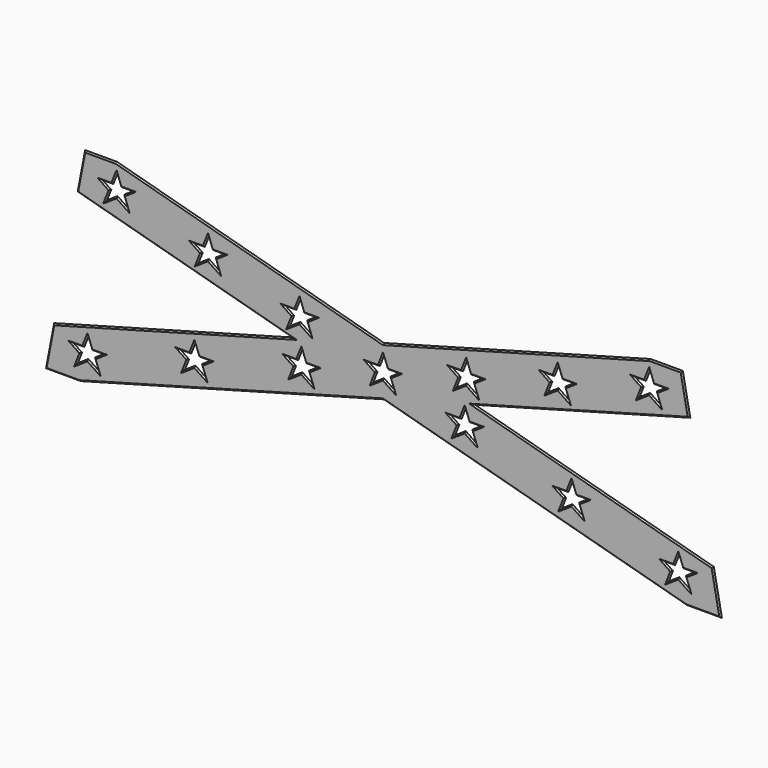
from build123d import *

# Parameters (mm, degrees)
F2_DEPTH = 3.175
F4_DEPTH = 3.175
F5_SIZE  = 3.17499


# Not quite as in the source:
# - a fillet or chamfer is up to 0.001 mm smaller than in the source, because OpenCascade refuses the exact size


with BuildPart() as f2:
    # F1 (on face) → F2 (new body)
    with BuildSketch(Plane.XZ):
        Polygon((-719.0774731079, 243.080791305), (-736.9299944829, 149.538113026), (-219.4252927257, 8.6387051816), (-793.6587311705, -147.7060607049), (-813.1201987879, -249.679208695), (-729.3418953294, -249.679208695), (0, -51.1035420022), (729.3418953294, -249.679208695), (813.1201987879, -249.679208695), (793.6587311705, -147.7060607049), (219.4252927257, 8.6387051816), (736.9299944829, 149.538113026), (719.0774731079, 243.080791305), (641.6491696493, 243.080791305), (0, 68.3809523654), (-641.6491696493, 243.080791305), align=None)
    extrude(amount=F2_DEPTH)

    # F3 (on face) → F4 (cut)
    with BuildSketch(Plane.XZ.offset(3.175)):
        Polygon((-641.1379151514, 218.6439759686), (-651.400474936, 193.2439759686), (-676.8718986419, 193.2439759686), (-656.2753553668, 179.4930621766), (-666.5379151514, 154.0930621766), (-641.1379151514, 171.0509179514), (-615.7379151514, 154.0930621766), (-625.1066068913, 179.4930621766), (-604.5100636162, 193.2439759686), (-631.7692234114, 193.2439759686), align=None)
        Polygon((-436.1568656837, 117.8018107739), (-446.4194254683, 92.4018107739), (-421.0194254683, 109.3596665488), (-395.6194254683, 92.4018107739), (-404.9881172082, 117.8018107739), (-384.3915739331, 131.552724566), (-411.6507337283, 131.552724566), (-421.0194254683, 156.952724566), (-431.2819852529, 131.552724566), (-456.7534089588, 131.552724566), align=None)
        Polygon((-216.0383760005, 56.1105593713), (-226.3009357851, 30.7105593713), (-200.9009357851, 47.6684151461), (-175.5009357851, 30.7105593713), (-184.8696275251, 56.1105593713), (-164.27308425, 69.8614731634), (-191.5322440452, 69.8614731634), (-200.9009357851, 95.2614731634), (-211.1634955697, 69.8614731634), (-236.6349192756, 69.8614731634), align=None)
        Polygon((-711.1145656244, -149.2288072846), (-721.1456436459, -174.6288072846), (-747.0800308779, -174.6288072846), (-726.4834876028, -188.3797210767), (-736.5145656244, -213.7797210767), (-711.1145656244, -196.8218653018), (-685.7145656244, -213.7797210767), (-695.3147391274, -188.3797210766), (-674.7181958523, -174.6288072846), (-701.5143921214, -174.6288072846), align=None)
        Polygon((-428.2842273396, -144.0767015538), (-437.8844008426, -118.6767015538), (-417.2878575675, -104.9257877617), (-444.0840538366, -104.9257877617), (-453.6842273396, -79.5257877617), (-463.7153053612, -104.9257877617), (-489.6496925932, -104.9257877617), (-469.0531493181, -118.6767015538), (-479.0842273396, -144.0767015538), (-453.6842273396, -127.118845779), align=None)
        Polygon((-170.8538890549, -74.3736820309), (-180.4540625579, -48.9736820309), (-159.8575192828, -35.2227682388), (-186.6537155519, -35.2227682388), (-196.2538890549, -9.8227682388), (-206.2849670764, -35.2227682388), (-232.2193543084, -35.2227682388), (-211.6228110334, -48.9736820309), (-221.6538890549, -74.3736820309), (-196.2538890549, -57.4158262561), align=None)
        Polygon((640.5082475643, 218.4725383182), (630.4771695428, 193.0725383182), (604.5427823108, 193.0725383182), (625.1393255859, 179.3216245261), (615.1082475643, 153.9216245261), (640.5082475643, 170.879480301), (665.9082475643, 153.9216245261), (656.3080740613, 179.3216245261), (676.9046173364, 193.0725383182), (650.1084210673, 193.0725383182), align=None)
        Polygon((429.9398402361, 131.5602955144), (420.3396667331, 156.9602955144), (410.3085887116, 131.5602955144), (384.3742014796, 131.5602955144), (404.9707447547, 117.8093817223), (394.9396667331, 92.4093817223), (420.3396667331, 109.3672374971), (445.7396667331, 92.4093817223), (436.1394932301, 117.8093817223), (456.7360365052, 131.5602955144), align=None)
        Polygon((209.7712594049, 70.0480527105), (200.1710859019, 95.4480527105), (190.1400078803, 70.0480527105), (164.2056206483, 70.0480527105), (184.8021639234, 56.2971389185), (174.7710859019, 30.8971389185), (200.1710859019, 47.8549946933), (225.5710859019, 30.8971389185), (215.9709123989, 56.2971389185), (236.567455674, 70.0480527105), align=None)
        Polygon((710.6600432828, -149.1050558895), (700.6289652612, -174.5050558895), (674.6945780292, -174.5050558895), (695.2911213043, -188.2559696816), (685.2600432828, -213.6559696816), (710.6600432828, -196.6981139068), (736.0600432828, -213.6559696816), (726.4598697798, -188.2559696816), (747.0564130549, -174.5050558895), (720.2602167857, -174.5050558895), align=None)
        Polygon((453.6346539421, -125.516380054), (479.0346539421, -142.4742358288), (469.4344804391, -117.0742358288), (490.0310237142, -103.3233220367), (463.2348274451, -103.3233220367), (453.6346539421, -77.9233220367), (443.6035759206, -103.3233220367), (417.6691886886, -103.3233220367), (438.2657319637, -117.0742358288), (428.2346539421, -142.4742358288), align=None)
        Polygon((196.6092646015, -54.3346462011), (222.0092646015, -71.292501976), (212.4090910985, -45.892501976), (233.0056343736, -32.1415881839), (206.2094381045, -32.1415881839), (196.6092646015, -6.7415881839), (186.5781865799, -32.1415881839), (160.6437993479, -32.1415881839), (181.240342623, -45.892501976), (171.2092646015, -71.292501976), align=None)
        Polygon((0, 41.4396189737), (-9.6761868873, 16.0396189737), (-36.3203563878, 16.0396189737), (-15.7238131127, 2.2887051816), (-25.4, -23.1112948184), (0, -6.1534390436), (25.4, -23.1112948184), (15.4449353628, 2.2887051816), (36.0414786379, 16.0396189737), (9.9550646372, 16.0396189737), align=None)
    extrude(amount=-F4_DEPTH, mode=Mode.SUBTRACT)

    # F5 (size 3.175 in the source; OpenCascade refuses exactly that, so slightly less here)
    f5_edges = [f2.edges().sort_by_distance(p)[0] for p in [
        (771.231047, -3.175, -249.679209),
        (364.670948, -3.175, -150.391375),
        (803.389465, -3.175, -198.692635),
        (-364.670948, -3.175, -150.391375),
        (506.542012, -3.175, -69.533678),
        (-771.231047, -3.175, -249.679209),
        (478.177644, -3.175, 79.088409),
        (-803.389465, -3.175, -198.692635),
        (728.003734, -3.175, 196.309452),
        (-506.542012, -3.175, -69.533678),
        (680.363321, -3.175, 243.080791),
        (-478.177644, -3.175, 79.088409),
        (320.824585, -3.175, 155.730872),
        (-728.003734, -3.175, 196.309452),
        (-320.824585, -3.175, 155.730872),
        (-680.363321, -3.175, 243.080791),
        (-690.514652, -3.175, -201.079721),
        (-685.016467, -3.175, -181.504264),
        (-688.116294, -3.175, -174.628807),
        (-706.314479, -3.175, -161.928807),
        (-716.130105, -3.175, -161.928807),
        (-734.112837, -3.175, -174.628807),
        (-736.781759, -3.175, -181.504264),
        (-731.499027, -3.175, -201.079721),
        (-723.814566, -3.175, -205.300793),
        (-698.414566, -3.175, -205.300793),
        (-433.084314, -3.175, -131.376702),
        (-427.586129, -3.175, -111.801245),
        (-430.685956, -3.175, -104.925788),
        (-448.884141, -3.175, -92.225788),
        (-458.699766, -3.175, -92.225788),
        (-476.682499, -3.175, -104.925788),
        (-479.351421, -3.175, -111.801245),
        (-474.068688, -3.175, -131.376702),
        (-466.384227, -3.175, -135.597774),
        (-440.984227, -3.175, -135.597774),
        (-183.553889, -3.175, -65.894754),
        (-175.653976, -3.175, -61.673682),
        (-170.155791, -3.175, -42.098225),
        (-173.255617, -3.175, -35.222768),
        (-191.453802, -3.175, -22.522768),
        (-201.269428, -3.175, -22.522768),
        (-219.252161, -3.175, -35.222768),
        (-221.921083, -3.175, -42.098225),
        (-216.63835, -3.175, -61.673682),
        (-208.953889, -3.175, -65.894754),
        (705.644504, -3.175, -161.805056),
        (687.661772, -3.175, -174.505056),
        (684.99285, -3.175, -181.380513),
        (690.275582, -3.175, -200.95597),
        (697.960043, -3.175, -205.177042),
        (723.360043, -3.175, -205.177042),
        (731.259957, -3.175, -200.95597),
        (736.758141, -3.175, -181.380513),
        (733.658315, -3.175, -174.505056),
        (715.46013, -3.175, -161.805056),
        (440.934654, -3.175, -133.995308),
        (466.334654, -3.175, -133.995308),
        (474.234567, -3.175, -129.774236),
        (479.732752, -3.175, -110.198779),
        (476.632926, -3.175, -103.323322),
        (458.434741, -3.175, -90.623322),
        (448.619115, -3.175, -90.623322),
        (430.636382, -3.175, -103.323322),
        (427.96746, -3.175, -110.198779),
        (433.250193, -3.175, -129.774236),
        (183.909265, -3.175, -62.813574),
        (209.309265, -3.175, -62.813574),
        (217.209178, -3.175, -58.592502),
        (222.707363, -3.175, -39.017045),
        (219.607536, -3.175, -32.141588),
        (201.409351, -3.175, -19.441588),
        (191.593726, -3.175, -19.441588),
        (173.610993, -3.175, -32.141588),
        (170.942071, -3.175, -39.017045),
        (176.224804, -3.175, -58.592502),
        (22.998272, -3.175, 16.039619),
        (4.977532, -3.175, 28.739619),
        (-4.838093, -3.175, 28.739619),
        (-22.998272, -3.175, 16.039619),
        (-26.022085, -3.175, 9.164162),
        (-20.561907, -3.175, -10.411295),
        (-12.7, -3.175, -14.632367),
        (12.7, -3.175, -14.632367),
        (20.422468, -3.175, -10.411295),
        (25.743207, -3.175, 9.164162),
        (-221.169656, -3.175, 43.410559),
        (-213.600936, -3.175, 39.189487),
        (-188.200936, -3.175, 39.189487),
        (-180.185282, -3.175, 43.410559),
        (-174.571356, -3.175, 62.986016),
        (-177.902664, -3.175, 69.861473),
        (-196.21659, -3.175, 82.561473),
        (-206.032216, -3.175, 82.561473),
        (-223.899207, -3.175, 69.861473),
        (-226.336648, -3.175, 62.986016),
        (-441.288146, -3.175, 105.101811),
        (-433.719425, -3.175, 100.880739),
        (-408.319425, -3.175, 100.880739),
        (-400.303771, -3.175, 105.101811),
        (-394.689846, -3.175, 124.677268),
        (-398.021154, -3.175, 131.552725),
        (-416.33508, -3.175, 144.252725),
        (-426.150705, -3.175, 144.252725),
        (-444.017697, -3.175, 131.552725),
        (-446.455137, -3.175, 124.677268),
        (-646.269195, -3.175, 205.943976),
        (-664.136187, -3.175, 193.243976),
        (-666.573627, -3.175, 186.368519),
        (-661.406635, -3.175, 166.793062),
        (-653.837915, -3.175, 162.57199),
        (-628.437915, -3.175, 162.57199),
        (-620.422261, -3.175, 166.793062),
        (-614.808335, -3.175, 186.368519),
        (-618.139644, -3.175, 193.243976),
        (-636.453569, -3.175, 205.943976),
        (204.971173, -3.175, 82.748053),
        (195.155547, -3.175, 82.748053),
        (177.172814, -3.175, 70.048053),
        (174.503892, -3.175, 63.172596),
        (179.786625, -3.175, 43.597139),
        (187.471086, -3.175, 39.376067),
        (212.871086, -3.175, 39.376067),
        (220.770999, -3.175, 43.597139),
        (226.269184, -3.175, 63.172596),
        (223.169358, -3.175, 70.048053),
        (425.139753, -3.175, 144.260296),
        (415.324128, -3.175, 144.260296),
        (397.341395, -3.175, 131.560296),
        (394.672473, -3.175, 124.684839),
        (399.955206, -3.175, 105.109382),
        (407.639667, -3.175, 100.88831),
        (433.039667, -3.175, 100.88831),
        (440.93958, -3.175, 105.109382),
        (446.437765, -3.175, 124.684839),
        (443.337938, -3.175, 131.560296),
        (635.492709, -3.175, 205.772538),
        (617.509976, -3.175, 193.072538),
        (614.841054, -3.175, 186.197081),
        (620.123787, -3.175, 166.621625),
        (627.808248, -3.175, 162.400552),
        (653.208248, -3.175, 162.400552),
        (661.108161, -3.175, 166.621625),
        (666.606346, -3.175, 186.197081),
        (663.506519, -3.175, 193.072538),
        (645.308334, -3.175, 205.772538),
    ]]
    chamfer(f5_edges, length=F5_SIZE)


solid = f2.part
